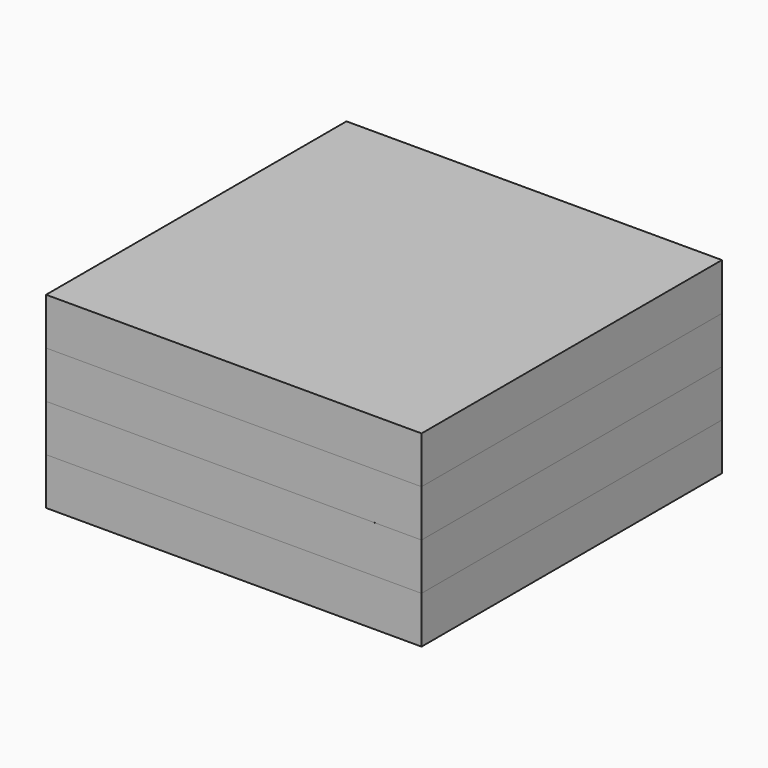
from build123d import *

# Parameters (mm, degrees)
F0_W     = 20
F0_H     = 20
F1_DEPTH = 2.5
F2_DEPTH = 2.5
F3_DEPTH = 2.5
F4_DEPTH = 2.5


with BuildPart() as f1:
    # F0 (on Top) → F1 (new body)
    with BuildSketch(Plane.XY):
        Rectangle(F0_W, F0_H)
    extrude(amount=F1_DEPTH)


with BuildPart() as f2:
    # F2 (new): a face of the model
    f2_faces = [f1.part.faces().sort_by_distance(p)[0] for p in [
        (0, 0, 2.5),
    ]]
    extrude(f2_faces, amount=F2_DEPTH)


with BuildPart() as f3:
    # F3 (new): a face of the model
    f3_faces = [f2.part.faces().sort_by_distance(p)[0] for p in [
        (0, 0, 5),
    ]]
    extrude(f3_faces, amount=F3_DEPTH)


with BuildPart() as f4:
    # F4 (new): a face of the model
    f4_faces = [f3.part.faces().sort_by_distance(p)[0] for p in [
        (0, 0, 7.5),
    ]]
    extrude(f4_faces, amount=F4_DEPTH)


solid = Compound([f1.part, f2.part, f3.part, f4.part])
